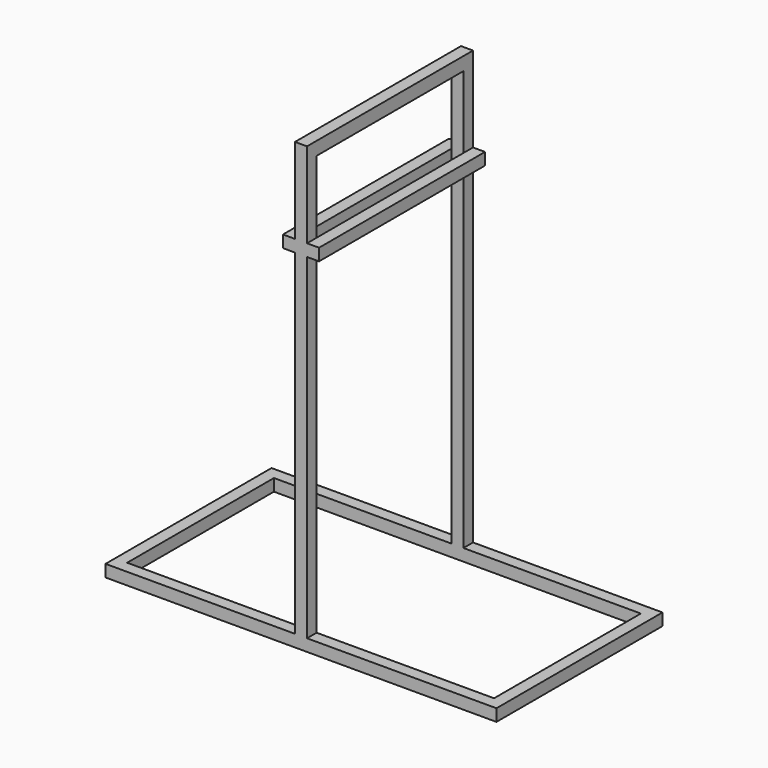
from build123d import *

# Parameters (mm, degrees)
F0_W      = 25.4
F0_H      = 25.4
F1_DEPTH  = 25.4
F0_H_2    = 387.35
F2_DEPTH  = 939.8
F4_DEPTH  = 25.4
F7_W      = 25.4
F7_H      = 25.4
F7_W_2    = 387.35
F8_DEPTH  = 25.4
F9_W      = 438.15
F9_H      = 25.4
F10_DEPTH = 25.4


# Not quite as in the source:
# - the program builds the solid bodies; features that only make, move or delete a surface that nothing else refers to are left out


with BuildPart() as f1:
    # F0 (on Top) → F1 (new body)
    with BuildSketch(Plane.XY):
        Polygon((412.75, -219.075), (412.75, 219.075), (38.1, 219.075), (38.1, 193.675), (387.35, 193.675), (387.35, -193.675), (38.1, -193.675), (38.1, -219.075), align=None)
        with Locations((25.4, 206.375)):
            Rectangle(F0_W, F0_H)
        with Locations((0, 206.375)):
            Rectangle(F0_W, F0_H)
        with Locations((25.4, -206.375)):
            Rectangle(F0_W, F0_H)
        with Locations((-25.4, 206.375)):
            Rectangle(F0_W, F0_H)
        with Locations((0, -206.375)):
            Rectangle(F0_W, F0_H)
        Polygon((-38.1, 193.675), (-38.1, 219.075), (-412.75, 219.075), (-412.75, -219.075), (-38.1, -219.075), (-38.1, -193.675), (-387.35, -193.675), (-387.35, 193.675), align=None)
        with Locations((-25.4, -206.375)):
            Rectangle(F0_W, F0_H)
    extrude(amount=F1_DEPTH)

    # F0 (on Top) → F2 (join)
    with BuildSketch(Plane.XY):
        Rectangle(F0_W, F0_H_2)
        with Locations((0, 206.375)):
            Rectangle(F0_W, F0_H)
        with Locations((0, -206.375)):
            Rectangle(F0_W, F0_H)
    extrude(amount=F2_DEPTH)

    # F3 (on face) → F4 (cut)
    with BuildSketch(Plane(origin=(-12.7, 0, 0), x_dir=(0, -1, 0), z_dir=(-1, 0, 0))):
        Polygon((-193.675, -2.54), (193.675, -2.54), (193.675, 737.5616856575), (193.675, 911.86), (-193.675, 911.86), (-193.675, 737.5616856575), align=None)
    extrude(amount=-F4_DEPTH, mode=Mode.SUBTRACT)

    # F7 (on face) → F8 (join)
    with BuildSketch(Plane(origin=(-12.7, 0, 0), x_dir=(0, -1, 0), z_dir=(-1, 0, 0))):
        with Locations((206.375, 746.76)):
            Rectangle(F7_W, F7_H)
        with Locations((0, 746.76)):
            Rectangle(F7_W_2, F7_H)
        with Locations((-206.375, 746.76)):
            Rectangle(F7_W, F7_H)
    extrude(amount=F8_DEPTH)

    # F9 (on face) → F10 (join)
    with BuildSketch(Plane.YZ.offset(12.7)):
        with Locations((0, 746.9166304588)):
            Rectangle(F9_W, F9_H)
    extrude(amount=F10_DEPTH)


solid = f1.part
